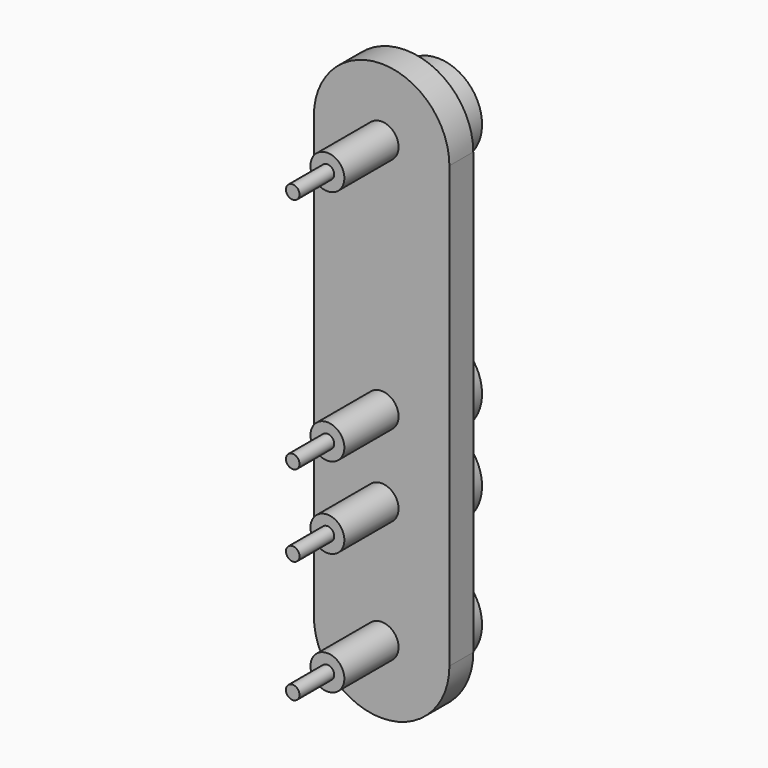
from build123d import *

# Parameters (mm, degrees)
F1_DEPTH = 5.588
F3_DEPTH = 7.62
F4_R     = 3.175
F5_DEPTH = 12.7
F6_R     = 1.27
F7_DEPTH = 8.128


with BuildPart() as f1:
    # F0 (on Front) → F1 (new body)
    with BuildSketch(Plane.XZ):
        with BuildLine():
            Line((12.7, -41.275), (12.7, 41.275))
            ThreePointArc((12.7, 41.275), (0, 53.975), (-12.7, 41.275))
            Line((-12.7, 41.275), (-12.7, -41.275))
            ThreePointArc((-12.7, -41.275), (0, -53.975), (12.7, -41.275))
        make_face()
    extrude(amount=F1_DEPTH)

    # F2 (on face) → F3 (join)
    with BuildSketch(Plane(origin=(0, 0, 0), x_dir=(-1, 0, 0), z_dir=(0, 1, 0))):
        with BuildLine():
            ThreePointArc((4.445, 34.3189235197), (7.2401139494, 37.309426271), (8.255, 41.275))
            ThreePointArc((8.255, 41.275), (-3.965573729, 48.5151139494), (-4.445, 34.3189235197))
            ThreePointArc((-4.445, 34.3189235197), (0, 33.02), (4.445, 34.3189235197))
        make_face()
        with BuildLine():
            ThreePointArc((4.445, 34.3189235197), (0, 33.02), (-4.445, 34.3189235197))
            Line((-4.445, 34.3189235197), (-4.445, 3.7810764803))
            ThreePointArc((-4.445, 3.7810764803), (0, 5.08), (4.445, 3.7810764803))
            Line((4.445, 3.7810764803), (4.445, 34.3189235197))
        make_face()
        with BuildLine():
            ThreePointArc((4.445, 3.7810764803), (0, 5.08), (-4.445, 3.7810764803))
            ThreePointArc((-4.445, 3.7810764803), (-8.2238434682, -3.89153584), (-3.175, -10.795))
            ThreePointArc((-3.175, -10.795), (0, -10.16), (3.175, -10.795))
            ThreePointArc((3.175, -10.795), (6.8685751798, -7.7540501198), (8.255, -3.175))
            ThreePointArc((8.255, -3.175), (7.2401139494, 0.790573729), (4.445, 3.7810764803))
        make_face()
        with BuildLine():
            ThreePointArc((3.175, -10.795), (0, -11.43), (-3.175, -10.795))
            ThreePointArc((-3.175, -10.795), (-8.2238434682, -17.69846416), (-4.445, -25.3710764803))
            ThreePointArc((-4.445, -25.3710764803), (0, -26.67), (4.445, -25.3710764803))
            ThreePointArc((4.445, -25.3710764803), (7.2401139494, -22.380573729), (8.255, -18.415))
            ThreePointArc((8.255, -18.415), (6.8685751798, -13.8359498802), (3.175, -10.795))
        make_face()
        with BuildLine():
            ThreePointArc((3.175, -10.795), (0, -10.16), (-3.175, -10.795))
            ThreePointArc((-3.175, -10.795), (0, -11.43), (3.175, -10.795))
        make_face()
        with BuildLine():
            ThreePointArc((4.445, -25.3710764803), (0, -26.67), (-4.445, -25.3710764803))
            Line((-4.445, -25.3710764803), (-4.445, -34.3189235197))
            ThreePointArc((-4.445, -34.3189235197), (0, -33.02), (4.445, -34.3189235197))
            Line((4.445, -34.3189235197), (4.445, -25.3710764803))
        make_face()
        with BuildLine():
            ThreePointArc((4.445, -34.3189235197), (0, -33.02), (-4.445, -34.3189235197))
            ThreePointArc((-4.445, -34.3189235197), (-3.965573729, -48.5151139494), (8.255, -41.275))
            ThreePointArc((8.255, -41.275), (7.2401139494, -37.309426271), (4.445, -34.3189235197))
        make_face()
    extrude(amount=F3_DEPTH)

    # F4 (on face) → F5 (join)
    with BuildSketch(Plane.XZ.offset(5.588)):
        with Locations((0, -41.275)):
            Circle(F4_R)
        with Locations((0, 41.275)):
            Circle(F4_R)
        with Locations((0, -3.175)):
            Circle(F4_R)
        with Locations((0, -18.415)):
            Circle(F4_R)
    extrude(amount=F5_DEPTH)

    # F6 (on face) → F7 (join)
    with BuildSketch(Plane.XZ.offset(18.288)):
        with Locations((0, 41.275)):
            Circle(F6_R)
        with Locations((0, -3.175)):
            Circle(F6_R)
        with Locations((0, -18.415)):
            Circle(F6_R)
        with Locations((0, -41.275)):
            Circle(F6_R)
    extrude(amount=F7_DEPTH)


solid = f1.part
